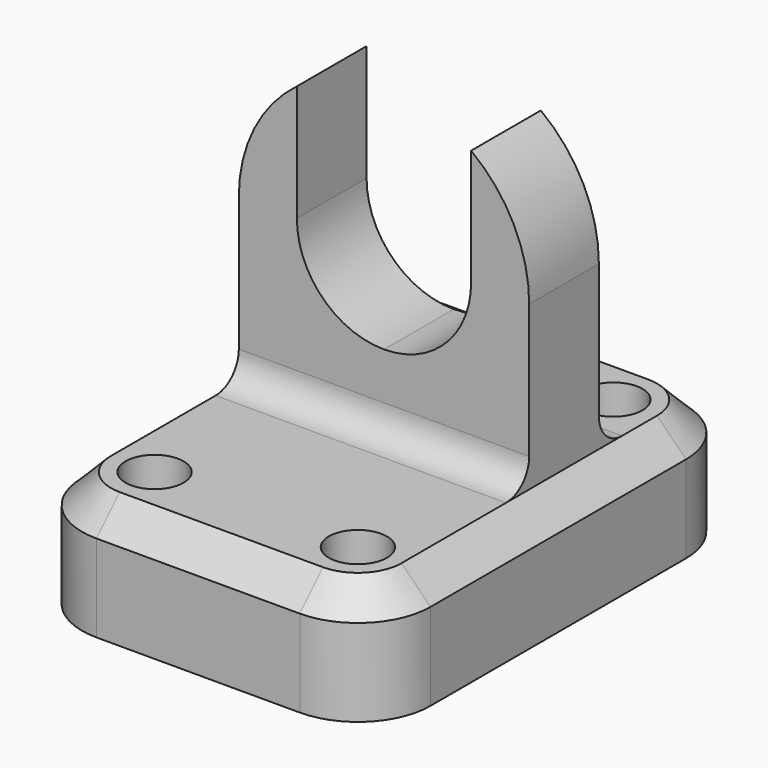
from build123d import *

# Parameters (mm, degrees)
F0_R     = 6.35
F1_DEPTH = 25.4
F2_SIZE  = 6.35
F3_W     = 63.5
F3_H     = 19.05
F4_DEPTH = 95.25
F5_R     = 6.35
F7_DEPTH = 50.801


with BuildPart() as f1:
    # F0 (on Top) → F1 (new body)
    with BuildSketch(Plane.XY):
        with BuildLine():
            ThreePointArc((0, 15.875), (4.6496798487, 4.6496798487), (15.875, 0))
            Line((15.875, 0), (60.325, 0))
            ThreePointArc((60.325, 0), (71.5503201513, 4.6496798487), (76.2, 15.875))
            Line((76.2, 15.875), (76.2, 85.725))
            ThreePointArc((76.2, 85.725), (71.5503201513, 96.9503201513), (60.325, 101.6))
            Line((60.325, 101.6), (15.875, 101.6))
            ThreePointArc((15.875, 101.6), (4.6496798487, 96.9503201513), (0, 85.725))
            Line((0, 85.725), (0, 15.875))
        make_face()
        with Locations((15.875, 15.875)):
            Circle(F0_R, mode=Mode.SUBTRACT)
        with Locations((60.325, 15.875)):
            Circle(F0_R, mode=Mode.SUBTRACT)
        with Locations((15.875, 85.725)):
            Circle(F0_R, mode=Mode.SUBTRACT)
        with Locations((60.325, 85.725)):
            Circle(F0_R, mode=Mode.SUBTRACT)
    extrude(amount=F1_DEPTH)

    # F2
    f2_edges = [f1.edges().sort_by_distance(p)[0] for p in [
        (38.1, 0, 25.4),
        (0, 50.8, 25.4),
        (4.64968, 4.64968, 25.4),
        (71.55032, 4.64968, 25.4),
        (76.2, 50.8, 25.4),
        (71.55032, 96.95032, 25.4),
        (38.1, 101.6, 25.4),
        (4.64968, 96.95032, 25.4),
    ]]
    chamfer(f2_edges, length=F2_SIZE)

    # F3 (on face) → F4 (join)
    with BuildSketch(Plane.XY.offset(25.4)):
        with Locations((38.1, 60.325)):
            Rectangle(F3_W, F3_H)
    extrude(amount=F4_DEPTH)

    # F5
    f5_edges = [f1.edges().sort_by_distance(p)[0] for p in [
        (38.1, 50.8, 25.4),
        (38.1, 69.85, 25.4),
    ]]
    fillet(f5_edges, radius=F5_R)

    # F6 (on face) → F7 (cut, through all)
    with BuildSketch(Plane.XZ.offset(-50.8)):
        with BuildLine():
            Line((6.35, 120.65), (6.35, 61.0775296334))
            ThreePointArc((6.35, 61.0775296334), (9.7019366858, 75.2765612905), (19.05, 86.4775296334))
            Line((19.05, 86.4775296334), (19.05, 120.65))
            Line((19.05, 120.65), (6.35, 120.65))
        make_face()
        with BuildLine():
            ThreePointArc((57.15, 61.0775296334), (38.1, 80.1275296334), (19.05, 61.0775296334))
            Line((19.05, 61.0775296334), (38.1, 61.0775296334))
            Line((38.1, 61.0775296334), (38.1, 42.0275296334))
            ThreePointArc((38.1, 42.0275296334), (51.5703841816, 47.6071454518), (57.15, 61.0775296334))
        make_face()
        with BuildLine():
            Line((19.05, 86.4775296334), (19.05, 61.0775296334))
            ThreePointArc((19.05, 61.0775296334), (38.1, 80.1275296334), (57.15, 61.0775296334))
            Line((57.15, 61.0775296334), (57.15, 86.4775296334))
            ThreePointArc((57.15, 86.4775296334), (38.1, 92.8275296334), (19.05, 86.4775296334))
        make_face()
        with BuildLine():
            Line((38.1, 61.0775296334), (19.05, 61.0775296334))
            ThreePointArc((19.05, 61.0775296334), (24.6296158184, 47.6071454518), (38.1, 42.0275296334))
            Line((38.1, 42.0275296334), (38.1, 61.0775296334))
        make_face()
        with BuildLine():
            Line((19.05, 120.65), (19.05, 86.4775296334))
            ThreePointArc((19.05, 86.4775296334), (38.1, 92.8275296334), (57.15, 86.4775296334))
            Line((57.15, 86.4775296334), (57.15, 120.65))
            Line((57.15, 120.65), (19.05, 120.65))
        make_face()
        with BuildLine():
            ThreePointArc((57.15, 86.4775296334), (66.4980633142, 75.2765612905), (69.85, 61.0775296334))
            Line((69.85, 61.0775296334), (69.85, 120.65))
            Line((69.85, 120.65), (57.15, 120.65))
            Line((57.15, 120.65), (57.15, 86.4775296334))
        make_face()
    extrude(amount=-F7_DEPTH, mode=Mode.SUBTRACT)


solid = f1.part
